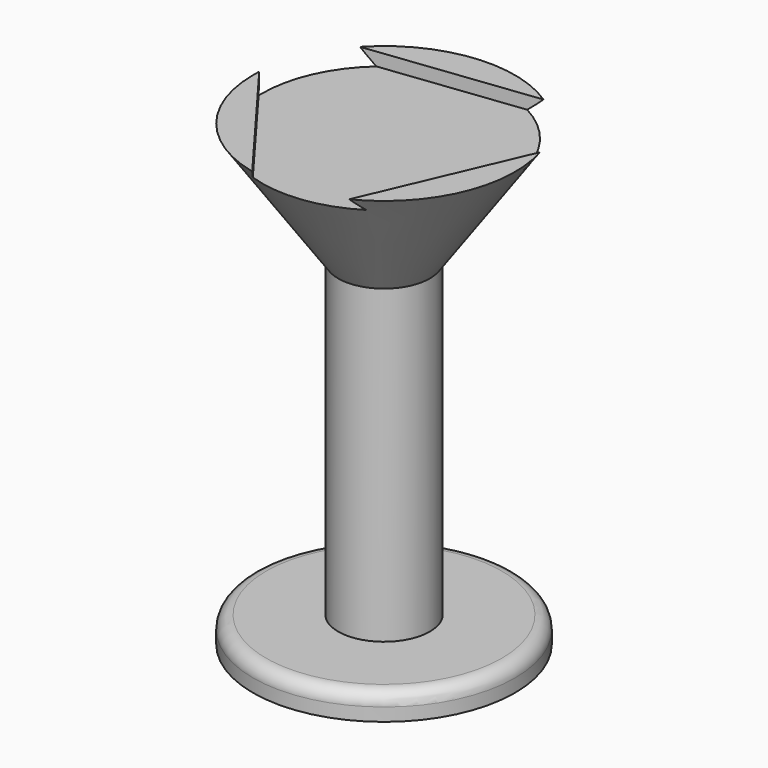
from build123d import *

# Parameters (mm, degrees)
F0_R     = 10
F1_DEPTH = 2
F3_R     = 1
F6_DEPTH = 1


with BuildPart() as f1:
    # F0 (on Top) → F1 (new body)
    with BuildSketch(Plane.XY):
        Circle(F0_R)
    extrude(amount=F1_DEPTH)

    # F3
    f3_edges = [f1.edges().sort_by_distance(p)[0] for p in [
        (-10, 0, 2),
    ]]
    fillet(f3_edges, radius=F3_R)

    # F2 (on Front) → F4 (revolve)
    with BuildSketch(Plane.XZ):
        Polygon((0, 35), (-10, 35), (-3.5, 25.7257949561), (-3.5, 2), (0, 2), align=None)
    revolve(axis=Axis((0, 0, 18.5), (0, 0, -1)))

    # F5 (on face) → F6 (cut)
    with BuildSketch(Plane.XY.offset(35)):
        Polygon((1.8076821121, -15.1926172437), (12.253351427, 9.1618072529), (-14.0610335391, 6.0308099908), align=None)
    extrude(amount=-F6_DEPTH, mode=Mode.SUBTRACT)


solid = f1.part
